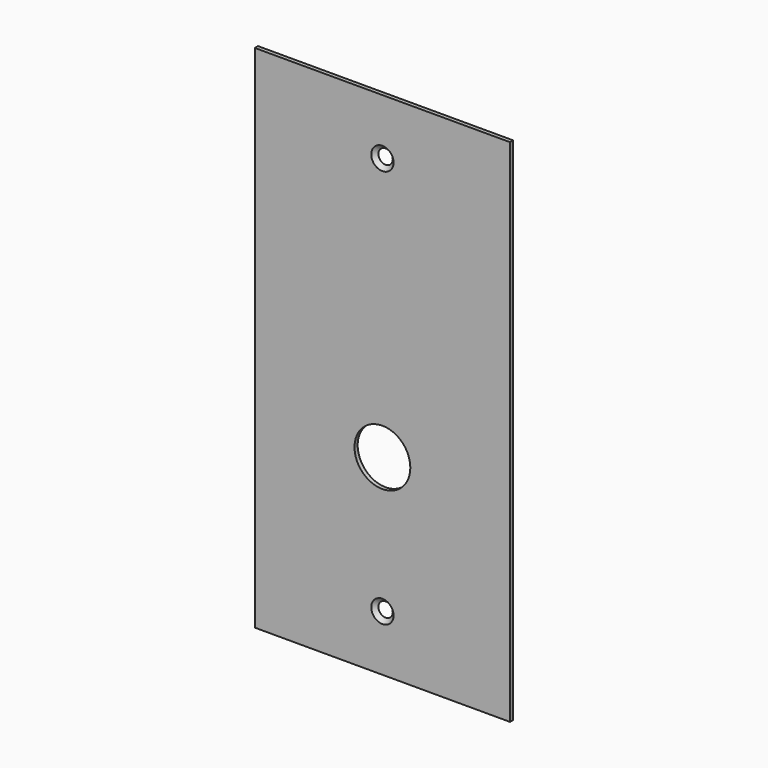
from build123d import *

# Parameters (mm, degrees)
F0_W     = 160
F0_H     = 320
F0_R     = 3
F0_R_2   = 17.5
F1_DEPTH = 2.5


# Not quite as in the source:
# - a fillet or chamfer that OpenCascade refuses, or shapes differently, is made with other operations: its cross-section is extruded or revolved along the edge and cut away or added


with BuildPart() as f1:
    # F0 (on Front) → F1 (new body)
    with BuildSketch(Plane.XZ):
        with Locations((-1.8876045942, 29.6809725389)):
            Rectangle(F0_W, F0_H)
        with Locations((-1.8876045942, -95.3190274611)):
            Circle(F0_R, mode=Mode.SUBTRACT)
        with Locations((-1.8876045942, -10.3190274611)):
            Circle(F0_R_2, mode=Mode.SUBTRACT)
        with Locations((-1.8876045942, 154.6809725389)):
            Circle(F0_R, mode=Mode.SUBTRACT)
    extrude(amount=F1_DEPTH)

    # F2: chamfer of 4 on 2 edges, made by hand

    # F2_s1 → F2_t2 (revolve, cut)
    with BuildSketch(Plane.XY.offset(154.6809725389)):
        Polygon((1.1123954058, 1.5), (5.1123954058, -2.5), (1.1123954058, -2.5), align=None)
    revolve(axis=Axis((-1.8876045942, -2.5, 154.6809725389), (0, -1, 0)), mode=Mode.SUBTRACT)

    # F2_s3 → F2_t4 (revolve, cut)
    with BuildSketch(Plane.XY.offset(-95.3190274611)):
        Polygon((1.1123954058, 1.5), (5.1123954058, -2.5), (1.1123954058, -2.5), align=None)
    revolve(axis=Axis((-1.8876045942, -2.5, -95.3190274611), (0, -1, 0)), mode=Mode.SUBTRACT)


solid = f1.part
